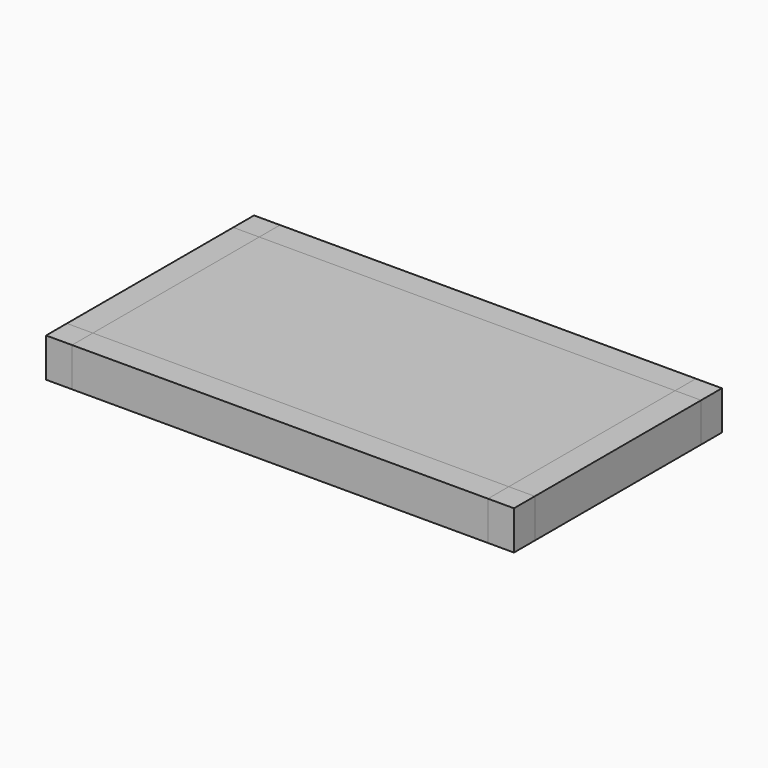
from build123d import *

# Parameters (mm, degrees)
F0_W      = 203.2
F0_H      = 101.6
F1_DEPTH  = 19.05
F2_W      = 12.7
F2_H      = 12.7
F3_DEPTH  = 19.05
F6_W      = 203.2
F6_H      = 12.7
F7_DEPTH  = 19.05
F9_W      = 12.7
F9_H      = 101.6
F10_DEPTH = 19.05


# Not quite as in the source:
# - a length typed as a fraction of an inch, garbled in the dataset ("3 / 203.2 mm" for 3/8 in), is restored


with BuildPart() as f1:
    # F0 (on Top) → F1 (new body)
    with BuildSketch(Plane.XY):
        Rectangle(F0_W, F0_H)
    extrude(amount=F1_DEPTH)


with BuildPart() as f3:
    # F2 (on face) → F3 (new body)
    with BuildSketch(Plane.XY.offset(19.05)):
        with Locations((-107.95, -57.15)):
            Rectangle(F2_W, F2_H)
    extrude(amount=-F3_DEPTH)


with BuildPart() as f4_1:
    # F4: instance of F3
    add(f3.part.mirror(Plane.YZ))


with BuildPart() as f5_1:
    # F5: instance of F3
    add(f3.part.mirror(Plane.XZ))


with BuildPart() as f5_2:
    # F5: instance of F4_1
    add(f4_1.part.mirror(Plane.XZ))


with BuildPart() as f7:
    # F6 (on face) → F7 (new body)
    with BuildSketch(Plane.XY.offset(19.05)):
        with Locations((0, -57.15)):
            Rectangle(F6_W, F6_H)
    extrude(amount=-F7_DEPTH)


with BuildPart() as f8_1:
    # F8: instance of F7
    add(f7.part.mirror(Plane.XZ))


with BuildPart() as f10:
    # F9 (on face) → F10 (new body)
    with BuildSketch(Plane.XY.offset(19.05)):
        with Locations((-107.95, 0)):
            Rectangle(F9_W, F9_H)
    extrude(amount=-F10_DEPTH)


with BuildPart() as f11_1:
    # F11: instance of F10
    add(f10.part.mirror(Plane.YZ))


solid = Compound([f1.part, f3.part, f4_1.part, f5_1.part, f5_2.part, f7.part, f8_1.part, f10.part, f11_1.part])
